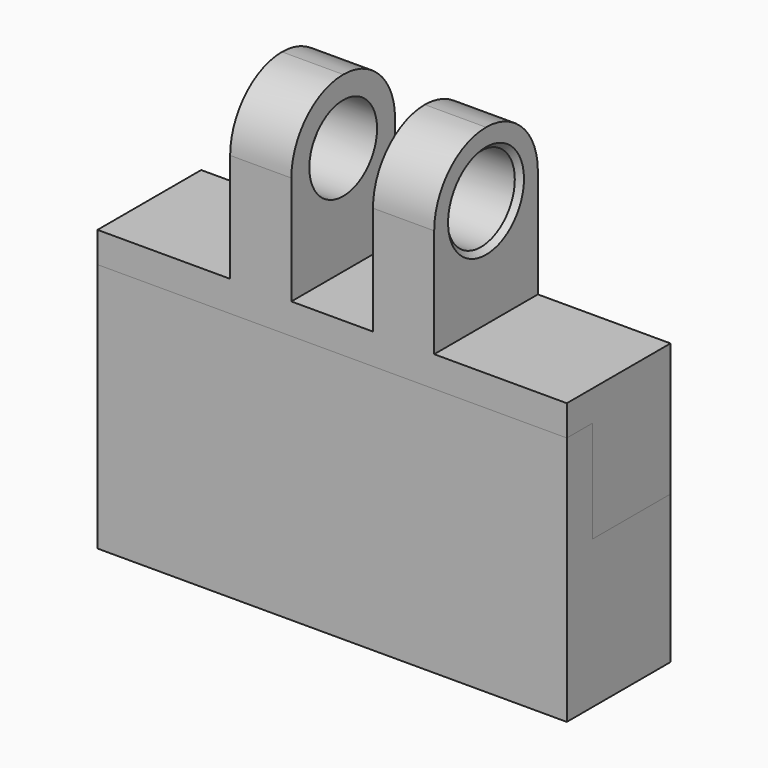
from build123d import *

# Parameters (mm, degrees)
F0_W          = 5.4
F0_H          = 9.55
F0_W_2        = 35.2
F0_H_2        = 3.15
F1_DEPTH      = 12.25
F4_START      = -2
F3_W          = 6
F3_H          = 12.7
F3_W_2        = 8
F3_W_3        = 5.4
F3_H_2        = 9.55
F4_DEPTH      = 3
F5_START      = -2
F5_DEPTH      = 13
F6_DEPTH      = 15
F6_DEPTH_BACK = 2
F7_R          = 4.15
F8_DEPTH      = 25
F9_R          = 6.34999
F10_SIZE      = 0.5


# Not quite as in the source:
# - a fillet or chamfer is up to 0.001 mm smaller than in the source, because OpenCascade refuses the exact size


with BuildPart() as f1:
    # F0 (on Top) → F1 (new body, symmetric)
    with BuildSketch(Plane.XY):
        with Locations((-20.3, 1.575)):
            Rectangle(F0_W, F0_H)
        with Locations((0, 1.575)):
            Rectangle(F0_W_2, F0_H)
        with Locations((20.3, 1.575)):
            Rectangle(F0_W, F0_H)
        with Locations((20.3, -4.775)):
            Rectangle(F0_W, F0_H_2)
        with Locations((0, -4.775)):
            Rectangle(F0_W_2, F0_H_2)
        with Locations((-20.3, -4.775)):
            Rectangle(F0_W, F0_H_2)
    extrude(amount=F1_DEPTH, both=True)


with BuildPart() as f4:
    # F3 (on offset) → F4 (new body)
    with BuildSketch(Plane.XY.offset(17.25).offset(F4_START)):
        Polygon((10, 6.35), (10, -6.35), (23, -6.35), (23, -3.2), (17.6, -3.2), (17.6, 6.35), align=None)
        with Locations((7, 0)):
            Rectangle(F3_W, F3_H)
        Rectangle(F3_W_2, F3_H)
        with Locations((-7, 0)):
            Rectangle(F3_W, F3_H)
        Polygon((-23, -3.2), (-23, -6.35), (-10, -6.35), (-10, 6.35), (-17.6, 6.35), (-17.6, -3.2), align=None)
        with Locations((-20.3, 1.575)):
            Rectangle(F3_W_3, F3_H_2)
        with Locations((20.3, 1.575)):
            Rectangle(F3_W_3, F3_H_2)
    extrude(amount=-F4_DEPTH)

    # F3 (on offset) → F5 (join)
    with BuildSketch(Plane.XY.offset(17.25).offset(F5_START)):
        with Locations((20.3, 1.575)):
            Rectangle(F3_W_3, F3_H_2)
        with Locations((-20.3, 1.575)):
            Rectangle(F3_W_3, F3_H_2)
    extrude(amount=-F5_DEPTH)

    # F3 (on offset) → F6 (join, two sides)
    with BuildSketch(Plane.XY.offset(17.25)) as f6_sk:
        with Locations((7, 0)):
            Rectangle(F3_W, F3_H)
        with Locations((-7, 0)):
            Rectangle(F3_W, F3_H)
    extrude(amount=F6_DEPTH)
    extrude(f6_sk.sketch, amount=-F6_DEPTH_BACK)

    # F7 (on face) → F8 (cut)
    with BuildSketch(Plane.YZ.offset(10)):
        with Locations((0, 25.9)):
            Circle(F7_R)
    extrude(amount=-F8_DEPTH, mode=Mode.SUBTRACT)

    # F9 (radius 6.35 in the source; OpenCascade refuses exactly that, so slightly less here)
    f9_edges = [f4.edges().sort_by_distance(p)[0] for p in [
        (-7, 6.35, 32.25),
        (7, 6.35, 32.25),
        (-7, -6.35, 32.25),
        (7, -6.35, 32.25),
    ]]
    fillet(f9_edges, radius=F9_R)

    # F10
    f10_edges = [f4.edges().sort_by_distance(p)[0] for p in [
        (-10, -4.15, 25.9),
        (10, -4.15, 25.9),
    ]]
    chamfer(f10_edges, length=F10_SIZE)


solid = Compound([f1.part, f4.part])
